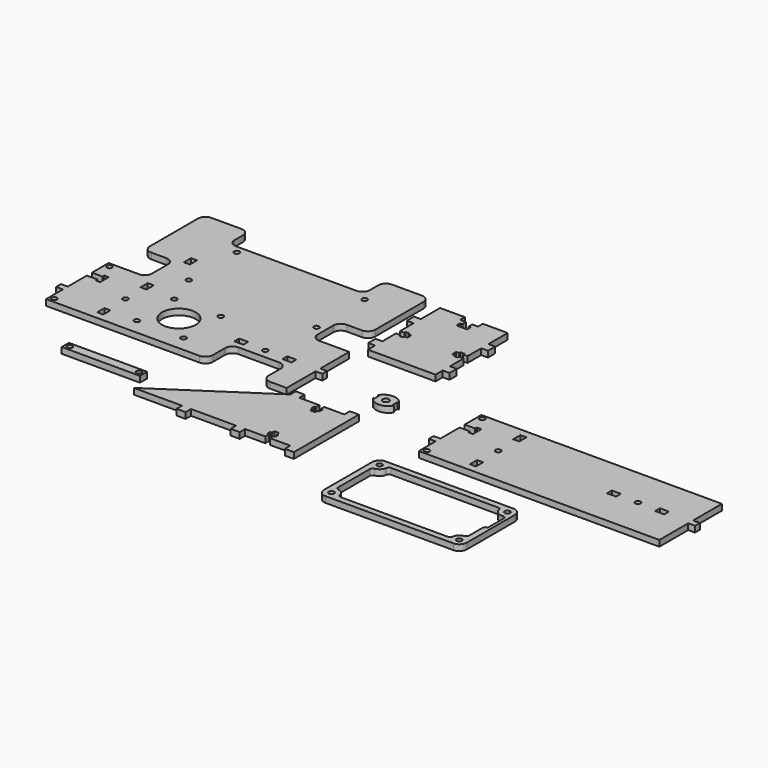
from build123d import *

# Parameters (mm, degrees)
F0_R     = 1.75
F0_W     = 4
F0_H     = 6
F0_R_2   = 11.25
F0_W_2   = 6
F0_H_2   = 4
F1_DEPTH = 4
F0_W_3   = 52
F0_R_3   = 2.1


# Not quite as in the source:
# - ends of sketch curves that miss each other by under 0.0002 mm in the source are joined


with BuildPart() as f1:
    # F0 (on Top) → F1 (new body)
    with BuildSketch(Plane.XY):
        with BuildLine():
            Line((-188.955769, 30.685527), (-208.955769, 30.685527))
            Line((-208.955769, 30.685527), (-208.955769, 16.785527))
            Line((-208.955769, 16.785527), (-201.955769, 16.785527))
            Line((-201.955769, 16.785527), (-201.955769, 18.235527))
            Line((-201.955769, 18.235527), (-198.955769, 18.235527))
            Line((-198.955769, 18.235527), (-198.955769, 11.135527))
            Line((-198.955769, 11.135527), (-201.955769, 11.135527))
            Line((-201.955769, 11.135527), (-201.955769, 12.585527))
            Line((-201.955769, 12.585527), (-208.955769, 12.585527))
            Line((-208.955769, 12.585527), (-208.955769, -3.314473))
            Line((-208.955769, -3.314473), (-213.455769, -3.314473))
            Line((-213.455769, -3.314473), (-213.455769, -7.314473))
            Line((-213.455769, -7.314473), (-208.955769, -7.314473))
            Line((-208.955769, -7.314473), (-208.955769, -21.314473))
            Line((-208.955769, -21.314473), (-106.955769, -21.314473))
            ThreePointArc((-106.955769, -21.314473), (-103.4202350941, -19.8500069059), (-101.955769, -16.314473))
            Line((-101.955769, -16.314473), (-101.955769, -6.314473))
            ThreePointArc((-101.955769, -6.314473), (-100.4913029059, -2.7789390941), (-96.955769, -1.314473))
            Line((-96.955769, -1.314473), (-69.955769, -1.314473))
            ThreePointArc((-69.955769, -1.314473), (-66.4202350941, -2.7789390941), (-64.955769, -6.314473))
            Line((-64.955769, -6.314473), (-64.955769, -16.314473))
            ThreePointArc((-64.955769, -16.314473), (-63.4913029059, -19.8500069059), (-59.955769, -21.314473))
            Line((-59.955769, -21.314473), (-48.955769, -21.314473))
            Line((-48.955769, -21.314473), (-48.955769, 2.685527))
            Line((-48.955769, 2.685527), (-44.455769, 2.685527))
            Line((-44.455769, 2.685527), (-44.455769, 6.685527))
            Line((-44.455769, 6.685527), (-48.955769, 6.685527))
            Line((-48.955769, 6.685527), (-48.955769, 30.685527))
            Line((-48.955769, 30.685527), (-68.955769, 30.685527))
            ThreePointArc((-68.955769, 30.685527), (-72.4913029059, 32.1499930941), (-73.955769, 35.685527))
            Line((-73.955769, 35.685527), (-73.955769, 48.685527))
            ThreePointArc((-73.955769, 48.685527), (-72.4913029059, 52.2210609059), (-68.955769, 53.685527))
            Line((-68.955769, 53.685527), (-58.955769, 53.685527))
            ThreePointArc((-58.955769, 53.685527), (-55.4202350941, 55.1499930941), (-53.955769, 58.685527))
            Line((-53.955769, 58.685527), (-53.955769, 98.685527))
            ThreePointArc((-53.955769, 98.685527), (-55.4202350941, 102.2210609059), (-58.955769, 103.685527))
            Line((-58.955769, 103.685527), (-78.955769, 103.685527))
            ThreePointArc((-78.955769, 103.685527), (-82.4913029059, 102.2210609059), (-83.955769, 98.685527))
            Line((-83.955769, 98.685527), (-83.955769, 91.685527))
            ThreePointArc((-83.955769, 91.685527), (-85.4202350941, 88.1499930941), (-88.955769, 86.685527))
            Line((-88.955769, 86.685527), (-168.955769, 86.685527))
            ThreePointArc((-168.955769, 86.685527), (-172.4913029059, 88.1499930941), (-173.955769, 91.685527))
            Line((-173.955769, 91.685527), (-173.955769, 98.685527))
            ThreePointArc((-173.955769, 98.685527), (-175.4202350941, 102.2210609059), (-178.955769, 103.685527))
            Line((-178.955769, 103.685527), (-198.955769, 103.685527))
            ThreePointArc((-198.955769, 103.685527), (-202.4913029059, 102.2210609059), (-203.955769, 98.685527))
            Line((-203.955769, 98.685527), (-203.955769, 58.685527))
            ThreePointArc((-203.955769, 58.685527), (-202.4913029059, 55.1499930941), (-198.955769, 53.685527))
            Line((-198.955769, 53.685527), (-188.955769, 53.685527))
            ThreePointArc((-188.955769, 53.685527), (-185.4202350941, 52.2210609059), (-183.955769, 48.685527))
            Line((-183.955769, 48.685527), (-183.955769, 35.685527))
            ThreePointArc((-183.955769, 35.685527), (-185.4202350941, 32.1499930941), (-188.955769, 30.685527))
        make_face()
        with Locations((-205.955769, -18.314473)):
            Circle(F0_R, mode=Mode.SUBTRACT)
        with Locations((-176.955769, -13.314473)):
            Rectangle(F0_W, F0_H, mode=Mode.SUBTRACT)
        with Locations((-156.955769, -10.814473)):
            Circle(F0_R, mode=Mode.SUBTRACT)
        with Locations((-125.955769, -10.814473)):
            Circle(F0_R, mode=Mode.SUBTRACT)
        with Locations((-176.955769, 4.685527)):
            Circle(F0_R, mode=Mode.SUBTRACT)
        with Locations((-176.955769, 22.685527)):
            Rectangle(F0_W, F0_H, mode=Mode.SUBTRACT)
        with Locations((-141.455769, 4.685527)):
            Circle(F0_R_2, mode=Mode.SUBTRACT)
        with Locations((-156.955769, 20.185527)):
            Circle(F0_R, mode=Mode.SUBTRACT)
        with Locations((-125.955769, 20.185527)):
            Circle(F0_R, mode=Mode.SUBTRACT)
        with Locations((-205.955769, 27.685527)):
            Circle(F0_R, mode=Mode.SUBTRACT)
        with Locations((-164.455769, 41.685527)):
            Circle(F0_R, mode=Mode.SUBTRACT)
        with Locations((-99.955769, 4.685527)):
            Rectangle(F0_W_2, F0_H_2, mode=Mode.SUBTRACT)
        with Locations((-83.955769, 4.685527)):
            Circle(F0_R, mode=Mode.SUBTRACT)
        with Locations((-67.955769, 4.685527)):
            Rectangle(F0_W_2, F0_H_2, mode=Mode.SUBTRACT)
        with Locations((-79.455769, 41.685527)):
            Circle(F0_R, mode=Mode.SUBTRACT)
        with Locations((-176.955769, 58.685527)):
            Rectangle(F0_W, F0_H, mode=Mode.SUBTRACT)
        with Locations((-164.455769, 81.685527)):
            Circle(F0_R, mode=Mode.SUBTRACT)
        with Locations((-79.455769, 81.685527)):
            Circle(F0_R, mode=Mode.SUBTRACT)
    extrude(amount=F1_DEPTH)


with BuildPart() as f1b:
    # F0 (on Top) → F1, piece 2 (new body)
    with BuildSketch(Plane.XY):
        with Locations((-142.955769, -55.314473)):
            Rectangle(F0_W_3, F0_H)
        with Locations((-165.955769, -55.314473)):
            Circle(F0_R, mode=Mode.SUBTRACT)
        with Locations((-119.955769, -55.314473)):
            Circle(F0_R, mode=Mode.SUBTRACT)
    extrude(amount=F1_DEPTH)


with BuildPart() as f1c:
    # F0 (on Top) → F1, piece 3 (new body)
    with BuildSketch(Plane.XY):
        Polygon((-6.955769, -75.314473), (-0.955769, -75.314473), (-0.955769, -21.314473), (-6.955769, -21.314473), (-6.955769, -25.814473), (-20.355769, -25.814473), (-20.355769, -28.814473), (-19.205769, -28.814473), (-19.205769, -31.414473), (-20.355769, -31.414473), (-20.355769, -33.414473), (-23.555769, -33.414473), (-23.555769, -31.414473), (-24.705769, -31.414473), (-24.705769, -28.814473), (-23.555769, -28.814473), (-23.555769, -25.814473), (-36.955769, -25.814473), (-36.955769, -21.314473), (-42.955769, -21.314473), (-42.955769, -25.814473), (-110.955769, -70.814473), (-78.955769, -70.814473), (-78.955769, -75.314473), (-72.955769, -75.314473), (-72.955769, -70.814473), (-42.955769, -70.814473), (-42.955769, -75.314473), (-36.955769, -75.314473), (-36.955769, -70.814473), (-23.555769, -70.814473), (-23.555769, -67.814473), (-24.705769, -67.814473), (-24.705769, -65.214473), (-23.555769, -65.214473), (-23.555769, -63.214473), (-20.355769, -63.214473), (-20.355769, -65.214473), (-19.205769, -65.214473), (-19.205769, -67.814473), (-20.355769, -67.814473), (-20.355769, -70.814473), (-6.955769, -70.814473), align=None)
    extrude(amount=F1_DEPTH)


with BuildPart() as f1d:
    # F0 (on Top) → F1, piece 4 (new body)
    with BuildSketch(Plane.XY):
        Polygon((-42.955769, 82.685527), (-47.455769, 82.685527), (-47.455769, 76.685527), (-42.955769, 76.685527), (-42.955769, 65.285527), (-39.955769, 65.285527), (-39.955769, 66.435527), (-37.355769, 66.435527), (-37.355769, 65.285527), (-35.355769, 65.285527), (-35.355769, 62.085527), (-37.355769, 62.085527), (-37.355769, 60.935527), (-39.955769, 60.935527), (-39.955769, 62.085527), (-42.955769, 62.085527), (-42.955769, 50.685527), (-47.455769, 50.685527), (-47.455769, 44.685527), (-42.955769, 44.685527), (-42.955769, 38.685527), (2.044231, 38.685527), (2.044231, 44.685527), (6.544231, 44.685527), (6.544231, 50.685527), (2.044231, 50.685527), (2.044231, 62.085527), (-0.955769, 62.085527), (-0.955769, 60.935527), (-3.555769, 60.935527), (-3.555769, 62.085527), (-5.555769, 62.085527), (-5.555769, 65.285527), (-3.555769, 65.285527), (-3.555769, 66.435527), (-0.955769, 66.435527), (-0.955769, 65.285527), (2.044231, 65.285527), (2.044231, 76.685527), (6.544231, 76.685527), (6.544231, 82.685527), (2.044231, 82.685527), (2.044231, 98.685527), (-14.455769, 98.685527), (-14.455769, 94.685527), (-18.355769, 94.685527), (-18.355769, 91.685527), (-16.905769, 91.685527), (-16.905769, 88.685527), (-24.005769, 88.685527), (-24.005769, 91.685527), (-22.555769, 91.685527), (-22.555769, 94.685527), (-26.455769, 94.685527), (-26.455769, 98.685527), (-42.955769, 98.685527), align=None)
    extrude(amount=F1_DEPTH)


with BuildPart() as f1e:
    # F0 (on Top) → F1, piece 5 (new body)
    with BuildSketch(Plane.XY):
        Polygon((55.955768, 0.04262), (48.955768, 0.04262), (48.955768, -15.85738), (44.455768, -15.85738), (44.455768, -19.85738), (48.955768, -19.85738), (48.955768, -33.85738), (208.955768, -33.85738), (208.955768, -9.85738), (213.455768, -9.85738), (213.455768, -5.85738), (208.955768, -5.85738), (208.955768, 18.14262), (48.955768, 18.14262), (48.955768, 4.24262), (55.955768, 4.24262), (55.955768, 5.69262), (58.955768, 5.69262), (58.955768, -1.40738), (55.955768, -1.40738), align=None)
        with Locations((51.955768, -30.85738)):
            Circle(F0_R, mode=Mode.SUBTRACT)
        with Locations((80.955768, -25.85738)):
            Rectangle(F0_W, F0_H, mode=Mode.SUBTRACT)
        with Locations((80.955768, -7.85738)):
            Circle(F0_R, mode=Mode.SUBTRACT)
        with Locations((157.955768, -7.85738)):
            Rectangle(F0_W_2, F0_H_2, mode=Mode.SUBTRACT)
        with Locations((173.955768, -7.85738)):
            Circle(F0_R, mode=Mode.SUBTRACT)
        with Locations((189.955768, -7.85738)):
            Rectangle(F0_W_2, F0_H_2, mode=Mode.SUBTRACT)
        with Locations((51.955768, 15.14262)):
            Circle(F0_R, mode=Mode.SUBTRACT)
        with Locations((80.955768, 10.14262)):
            Rectangle(F0_W, F0_H, mode=Mode.SUBTRACT)
    extrude(amount=F1_DEPTH)


with BuildPart() as f1f:
    # F0 (on Top) → F1, piece 6 (new body)
    with BuildSketch(Plane.XY):
        with BuildLine():
            Line((132.761374, -98.685527), (132.761374, -58.685527))
            ThreePointArc((132.761374, -58.685527), (131.2969079059, -55.1499930941), (127.761374, -53.685527))
            Line((127.761374, -53.685527), (42.761374, -53.685527))
            ThreePointArc((42.761374, -53.685527), (39.2258400941, -55.1499930941), (37.761374, -58.685527))
            Line((37.761374, -58.685527), (37.761374, -98.685527))
            ThreePointArc((37.761374, -98.685527), (39.2258400941, -102.2210609059), (42.761374, -103.685527))
            Line((42.761374, -103.685527), (127.761374, -103.685527))
            ThreePointArc((127.761374, -103.685527), (131.2969079059, -102.2210609059), (132.761374, -98.685527))
        make_face()
        with Locations((42.761374, -98.685527)):
            Circle(F0_R, mode=Mode.SUBTRACT)
        with BuildLine():
            ThreePointArc((43.4756599366, -63.634243561), (46.2969079059, -62.2210609059), (47.710090561, -59.3998129366))
            ThreePointArc((47.710090561, -59.3998129366), (48.3802695861, -58.1736691707), (49.689577, -57.685527))
            Line((49.689577, -57.685527), (120.833171, -57.685527))
            ThreePointArc((120.833171, -57.685527), (122.1424784679, -58.1736692175), (122.812657685, -59.3998130455))
            ThreePointArc((122.812657685, -59.3998130455), (124.7671794483, -62.6898745107), (128.4756599366, -63.634243561))
            ThreePointArc((128.4756599366, -63.634243561), (130.0706814139, -64.1018721707), (130.761374, -65.61373))
            Line((130.761374, -65.61373), (130.761374, -78.685527))
            ThreePointArc((130.761374, -78.685527), (129.3471604376, -79.2713134376), (128.761374, -80.685527))
            Line((128.761374, -80.685527), (128.761374, -91.757324))
            ThreePointArc((128.761374, -91.757324), (128.2732321532, -93.0666310398), (127.0470890755, -93.7368105232))
            ThreePointArc((127.0470890755, -93.7368105232), (124.2258404945, -95.1499926936), (122.8126574594, -97.971240922))
            ThreePointArc((122.8126574594, -97.971240922), (122.1424784679, -99.1973847825), (120.833171, -99.685527))
            Line((120.833171, -99.685527), (49.689577, -99.685527))
            ThreePointArc((49.689577, -99.685527), (48.3802695861, -99.1973848293), (47.7100903354, -97.9712410959))
            ThreePointArc((47.7100903354, -97.9712410959), (46.2969079059, -95.1499930941), (43.4756599366, -93.736810439))
            ThreePointArc((43.4756599366, -93.736810439), (42.2495161707, -93.0666314139), (41.761374, -91.757324))
            Line((41.761374, -91.757324), (41.761374, -65.61373))
            ThreePointArc((41.761374, -65.61373), (42.2495161707, -64.3044225861), (43.4756599366, -63.634243561))
        make_face(mode=Mode.SUBTRACT)
        with Locations((42.761374, -58.685527)):
            Circle(F0_R, mode=Mode.SUBTRACT)
        with Locations((127.761374, -98.685527)):
            Circle(F0_R, mode=Mode.SUBTRACT)
        with Locations((127.761374, -58.685527)):
            Circle(F0_R, mode=Mode.SUBTRACT)
    extrude(amount=F1_DEPTH)


with BuildPart() as f1g:
    # F0 (on Top) → F1, piece 7 (new body)
    with BuildSketch(Plane.XY):
        with BuildLine():
            ThreePointArc((7, 2), (0, 6), (-7, 2))
            Line((-7, 2), (-6, 2))
            Line((-6, 2), (-6, -2))
            Line((-6, -2), (-7, -2))
            ThreePointArc((-7, -2), (0, -6), (7, -2))
            Line((7, -2), (6, -2))
            Line((6, -2), (6, 2))
            Line((6, 2), (7, 2))
        make_face()
        Circle(F0_R_3, mode=Mode.SUBTRACT)
    extrude(amount=F1_DEPTH)


solid = Compound([f1.part, f1b.part, f1c.part, f1d.part, f1e.part, f1f.part, f1g.part])
